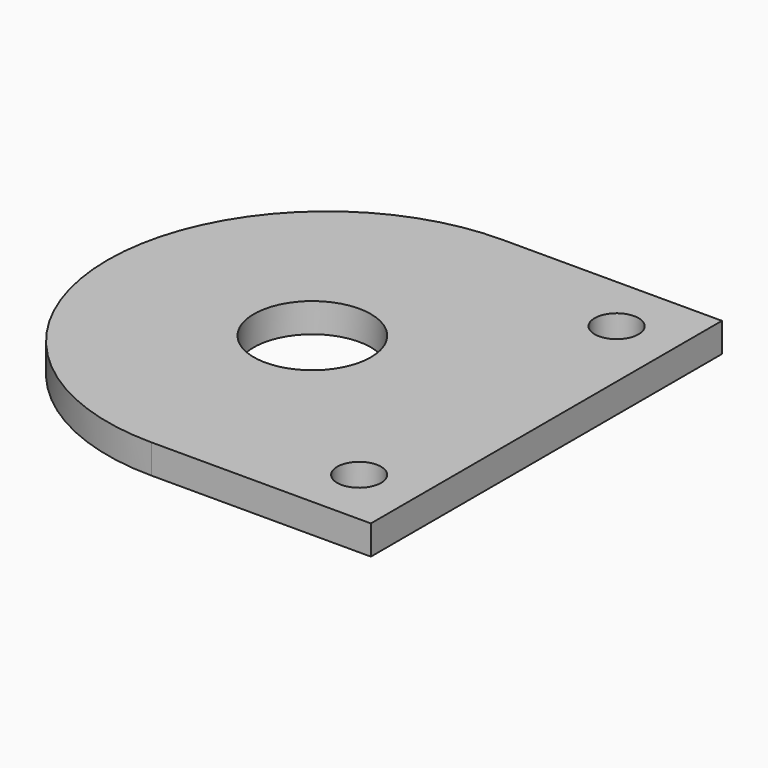
from build123d import *

# Parameters (mm, degrees)
F0_W     = 30
F0_H     = 30
F0_R     = 1.5
F0_R_2   = 4
F1_DEPTH = 2
F2_R     = 14.99999


# Not quite as in the source:
# - a fillet or chamfer is up to 0.001 mm smaller than in the source, because OpenCascade refuses the exact size


with BuildPart() as f1:
    # F0 (on Top) → F1 (new body)
    with BuildSketch(Plane.XY):
        with Locations((-15, 15)):
            Rectangle(F0_W, F0_H)
        with Locations((-4, 4)):
            Circle(F0_R, mode=Mode.SUBTRACT)
        with Locations((-16, 15)):
            Circle(F0_R_2, mode=Mode.SUBTRACT)
        with Locations((-4, 26)):
            Circle(F0_R, mode=Mode.SUBTRACT)
    extrude(amount=F1_DEPTH)

    # F2 (radius 15 in the source; OpenCascade refuses exactly that, so slightly less here)
    f2_edges = [f1.edges().sort_by_distance(p)[0] for p in [
        (-30, 0, 1),
        (-30, 30, 1),
    ]]
    fillet(f2_edges, radius=F2_R)


solid = f1.part
